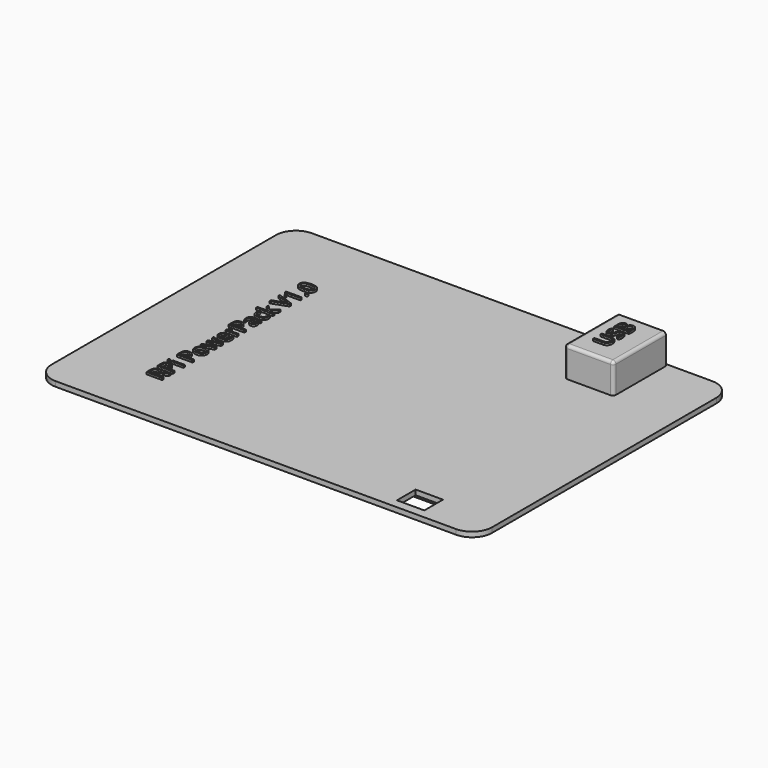
from build123d import *

# Parameters (mm, degrees)
F0_W          = 111.76
F0_H          = 81.28
F1_DEPTH      = 1.27
F2_R          = 5.08
F4_W          = 101.6
F4_H          = 58.42
F5_DEPTH      = 6.35
F6_R          = 5.08
F7_T1_DEPTH   = 1.27
F7_S5_W       = 5.1816
F7_S5_H       = 5.1816
F7_T6_DEPTH   = 5.1816
F7_S11_W      = 5.1816
F7_S11_H      = 5.1816
F7_T12_DEPTH  = 5.1816
F7_S17_W      = 5.1816
F7_S17_H      = 5.1816
F7_T18_DEPTH  = 5.1816
F7_S23_W      = 5.1816
F7_S23_H      = 5.1816
F7_T24_DEPTH  = 5.1816
F8_W          = 6.942614913
F8_H          = 5.9140771627
F9_DEPTH      = 5.08
F10_W         = 12.4787762761
F10_H         = 16.6547195404
F11_DEPTH     = 7.62
F12_TEXT_SIZE = 5.5671232877
F13_DEPTH     = 0.508
F14_R         = 0.762
F15_TEXT_SIZE = 5.2519182619
F16_DEPTH     = 0.508


# Not quite as in the source:
# - a fillet or chamfer that OpenCascade refuses, or shapes differently, is made with other operations: its cross-section is extruded or revolved along the edge and cut away or added
# - Text() gives the source's letters only with a copy of the font that has no kerning and outlines rounded to 1/6400 em; it was checked with that copy


with BuildPart() as f1:
    # F0 (on Top) → F1 (new body)
    with BuildSketch(Plane.XY):
        with Locations((55.88, -40.64)):
            Rectangle(F0_W, F0_H)
    extrude(amount=F1_DEPTH)

    # F2
    f2_edges = [f1.edges().sort_by_distance(p)[0] for p in [
        (111.76, -81.28, 0.635),
        (0, -81.28, 0.635),
        (111.76, 0, 0.635),
        (0, 0, 0.635),
    ]]
    fillet(f2_edges, radius=F2_R)

    # F4 (on face) → F5 (join)
    with BuildSketch(Plane(origin=(0, 0, 0), x_dir=(1, 0, 0), z_dir=(0, 0, -1))):
        with Locations((53.3387183125, 38.5634235731)):
            Rectangle(F4_W, F4_H)
    extrude(amount=F5_DEPTH)

    # F6
    f6_edges = [f1.edges().sort_by_distance(p)[0] for p in [
        (53.338718, -9.353424, -6.35),
        (2.538718, -38.563424, -6.35),
        (53.338718, -67.773424, -6.35),
        (104.138718, -38.563424, -6.35),
    ]]
    fillet(f6_edges, radius=F6_R)

    # F7: fillet of radius 5.08 on 8 edges, made by hand

    # F7_s2 → F7_t1 (cut)
    with BuildSketch(Plane.XY.offset(-1.27)):
        with BuildLine():
            ThreePointArc((2.5387183125, -62.6934235731), (4.0266158641, -66.2855260215), (7.6187183125, -67.7734235731))
            Line((7.6187183125, -67.7734235731), (2.5387183125, -67.7734235731))
            Line((2.5387183125, -67.7734235731), (2.5387183125, -62.6934235731))
        make_face()
        with BuildLine():
            ThreePointArc((2.5387183125, -14.4334235731), (4.0266158641, -10.8413211246), (7.6187183125, -9.3534235731))
            Line((7.6187183125, -9.3534235731), (2.5387183125, -9.3534235731))
            Line((2.5387183125, -9.3534235731), (2.5387183125, -14.4334235731))
        make_face()
        with BuildLine():
            ThreePointArc((99.0587183125, -67.7734235731), (102.6508207609, -66.2855260215), (104.1387183125, -62.6934235731))
            Line((104.1387183125, -62.6934235731), (104.1387183125, -67.7734235731))
            Line((104.1387183125, -67.7734235731), (99.0587183125, -67.7734235731))
        make_face()
        with BuildLine():
            ThreePointArc((99.0587183125, -9.3534235731), (102.6508207609, -10.8413211246), (104.1387183125, -14.4334235731))
            Line((104.1387183125, -14.4334235731), (104.1387183125, -9.3534235731))
            Line((104.1387183125, -9.3534235731), (99.0587183125, -9.3534235731))
        make_face()
    extrude(amount=F7_T1_DEPTH, mode=Mode.SUBTRACT)


with BuildPart() as f7_tool4:
    # F7_s5 → F7_t6 (new body)
    with BuildSketch(Plane.YZ.offset(7.6187183125)):
        with Locations((-65.2842235731, -3.8608)):
            Rectangle(F7_S5_W, F7_S5_H)
    extrude(amount=-F7_T6_DEPTH)

    # F7_s7 → F7_t8 (revolve, cut)
    with BuildSketch(Plane(origin=(7.6187183125, -62.6934235731, -1.27), x_dir=(0, 0.7071067812, 0.7071067812), z_dir=(0, -0.7071067812, 0.7071067812))):
        with BuildLine():
            ThreePointArc((0, -5.08), (5.08, 0), (0, 5.08))
            Line((0, 5.08), (0, -5.08))
        make_face()
    revolve(axis=Axis((7.6187183125, -62.6934235731, -1.27), (-1, 0, 0)), mode=Mode.SUBTRACT)


with BuildPart() as f1_1:
    add(f1.part)

    # F7_t3: cut F7_tool4
    add(f7_tool4.part, mode=Mode.SUBTRACT)


with BuildPart() as f7_tool10:
    # F7_s11 → F7_t12 (new body)
    with BuildSketch(Plane.XZ.offset(62.6934235731)):
        with Locations((101.6495183125, -3.8608)):
            Rectangle(F7_S11_W, F7_S11_H)
    extrude(amount=F7_T12_DEPTH)

    # F7_s13 → F7_t14 (revolve, cut)
    with BuildSketch(Plane(origin=(99.0587183125, -62.6934235731, -1.27), x_dir=(-0.7071067812, 0, 0.7071067812), z_dir=(0.7071067812, 0, 0.7071067812))):
        with BuildLine():
            ThreePointArc((0, -5.08), (5.08, 0), (0, 5.08))
            Line((0, 5.08), (0, -5.08))
        make_face()
    revolve(axis=Axis((99.0587183125, -62.6934235731, -1.27), (0, -1, 0)), mode=Mode.SUBTRACT)


with BuildPart() as f1_2:
    add(f1_1.part)

    # F7_t9: cut F7_tool10
    add(f7_tool10.part, mode=Mode.SUBTRACT)


with BuildPart() as f7_tool16:
    # F7_s17 → F7_t18 (new body)
    with BuildSketch(Plane.XZ.offset(14.4334235731)):
        with Locations((101.6495183125, -3.8608)):
            Rectangle(F7_S17_W, F7_S17_H)
    extrude(amount=-F7_T18_DEPTH)

    # F7_s19 → F7_t20 (revolve, cut)
    with BuildSketch(Plane(origin=(99.0587183125, -14.4334235731, -1.27), x_dir=(-0.7071067812, 0, 0.7071067812), z_dir=(-0.7071067812, 0, -0.7071067812))):
        with BuildLine():
            ThreePointArc((0, -5.08), (5.08, 0), (0, 5.08))
            Line((0, 5.08), (0, -5.08))
        make_face()
    revolve(axis=Axis((99.0587183125, -14.4334235731, -1.27), (0, 1, 0)), mode=Mode.SUBTRACT)


with BuildPart() as f1_3:
    add(f1_2.part)

    # F7_t15: cut F7_tool16
    add(f7_tool16.part, mode=Mode.SUBTRACT)


with BuildPart() as f7_tool22:
    # F7_s23 → F7_t24 (new body)
    with BuildSketch(Plane.YZ.offset(7.6187183125)):
        with Locations((-11.8426235731, -3.8608)):
            Rectangle(F7_S23_W, F7_S23_H)
    extrude(amount=-F7_T24_DEPTH)

    # F7_s25 → F7_t26 (revolve, cut)
    with BuildSketch(Plane(origin=(7.6187183125, -14.4334235731, -1.27), x_dir=(0, -0.7071067812, 0.7071067812), z_dir=(0, -0.7071067812, -0.7071067812))):
        with BuildLine():
            ThreePointArc((0, -5.08), (5.08, 0), (0, 5.08))
            Line((0, 5.08), (0, -5.08))
        make_face()
    revolve(axis=Axis((7.6187183125, -14.4334235731, -1.27), (-1, 0, 0)), mode=Mode.SUBTRACT)


with BuildPart() as f1_4:
    add(f1_3.part)

    # F7_t21: cut F7_tool22
    add(f7_tool22.part, mode=Mode.SUBTRACT)

    # F8 (on face) → F9 (cut)
    with BuildSketch(Plane.XY.offset(1.27)):
        with Locations((93.2929813862, -75.995914638)):
            Rectangle(F8_W, F8_H)
    extrude(amount=-F9_DEPTH, mode=Mode.SUBTRACT)

    # F10 (on face) → F11 (join)
    with BuildSketch(Plane.XY.offset(1.27)):
        with Locations((89.211601764, -8.9912438125)):
            Rectangle(F10_W, F10_H)
    extrude(amount=F11_DEPTH)

    # F12 (on face) → F13 (join)
    with BuildSketch(Plane.XY.offset(1.27)):
        with Locations(Location((21.275615975, -68.3026412528), (0, 0, 90))):
            Text('RPi PowerPack V1.0', F12_TEXT_SIZE, font='Open Sans', text_align=(TextAlign.LEFT, TextAlign.BOTTOM))
    extrude(amount=F13_DEPTH)

    # F14
    f14_edges = [f1_4.edges().sort_by_distance(p)[0] for p in [
        (82.972214, -8.991244, 8.89),
        (95.45099, -8.991244, 8.89),
        (89.211602, -17.318604, 8.89),
        (95.45099, -17.318604, 5.08),
        (82.972214, -17.318604, 5.08),
    ]]
    fillet(f14_edges, radius=F14_R)

    # F15 (on face) → F16 (join)
    with BuildSketch(Plane.XY.offset(8.89)):
        with Locations(Location((90.3374065111, -13.2255177992), (0, 0, 90))):
            Text('USB', F15_TEXT_SIZE, font='Open Sans', text_align=(TextAlign.LEFT, TextAlign.BOTTOM))
    extrude(amount=F16_DEPTH)


solid = f1_4.part
